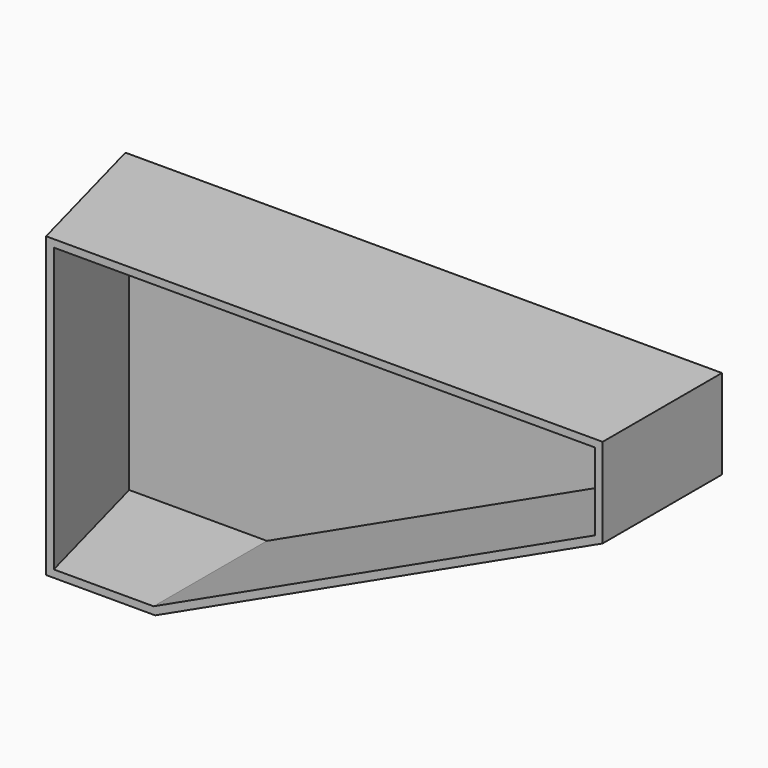
from build123d import *

# Parameters (mm, degrees)
F1_DEPTH = 50
F3_DEPTH = 100.001
F4_T     = -2.5


with BuildPart() as f1:
    # F0 (on Front) → F1 (new body)
    with BuildSketch(Plane.XZ):
        Polygon((100, 51.4285714286), (-100, 51.4285714286), (-100, -48.5714285714), (-50, -48.5714285714), (100, 21.4285714286), align=None)
    extrude(amount=F1_DEPTH)

    # F2 (on face) → F3 (cut, through all)
    with BuildSketch(Plane.XY.offset(51.4285714286)):
        Polygon((-121.3779896498, -70.3287050128), (-68.4581929454, -117.7156264903), (-86.6025403784, -50), (-100, -50), (-100, 0), (-122.3772391677, 0), align=None)
        Polygon((-100, -50), (-86.6025403784, -50), (-100, 0), align=None)
    extrude(amount=-F3_DEPTH, mode=Mode.SUBTRACT)

    # F4
    f4_openings = [f1.faces().sort_by_distance(p)[0] for p in [
        (-10.253348, -50, 11.868344),
    ]]
    offset(amount=F4_T, openings=f4_openings)


solid = f1.part
